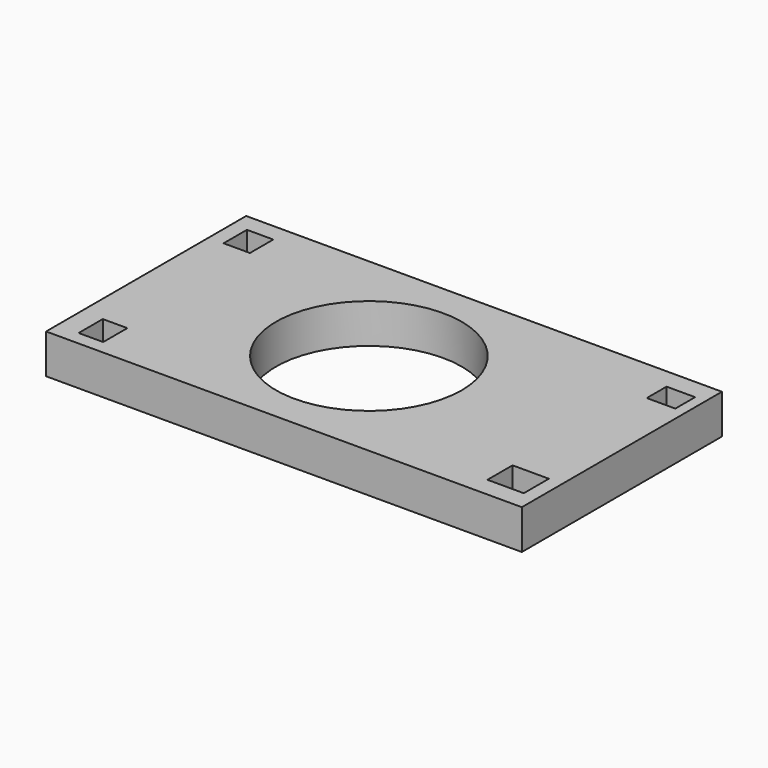
from build123d import *

# Parameters (mm, degrees)
F0_W      = 306.200504303
F0_H      = 160.9693467617
F1_DEPTH  = 25.4
F2_W      = 16.9635862112
F2_H      = 18.7774226069
F2_W_2    = 18.3757990599
F2_H_2    = 15.9212723374
F2_W_3    = 15.8156380057
F2_H_3    = 19.4401964545
F3_DEPTH  = 25.4
F4_W      = 23.3820155263
F4_H      = 20.1737955213
F5_DEPTH  = 25.4
F10_W     = 156.8522006273
F10_H     = 128.1716823578
F10_W_2   = 155.7295322418
F10_H_2   = 9.3674659729
F11_DEPTH = 25.4
F12_R     = 59.7527814568
F13_DEPTH = 25.4


# Not quite as in the source:
# - a feature of the source that left no trace in its solid (it failed there, or was rolled back) is left out


with BuildPart() as f1:
    # F0 (on Top) → F1 (new body)
    with BuildSketch(Plane.XY):
        Rectangle(F0_W, F0_H)
    extrude(amount=F1_DEPTH)

    # F2 (on face) → F3 (cut)
    with BuildSketch(Plane.XY.offset(25.4)):
        with Locations((-134.9064931273, 59.5765523612)):
            Rectangle(F2_W, F2_H)
        with Locations((137.0917782187, 59.4723559916)):
            Rectangle(F2_W_2, F2_H_2)
        with Locations((-131.3789226115, -61.8558935821)):
            Rectangle(F2_W_3, F2_H_3)
    extrude(amount=-F3_DEPTH, mode=Mode.SUBTRACT)

    # F4 (on face) → F5 (cut)
    with BuildSketch(Plane.XY.offset(25.4)):
        with Locations((132.6544694602, -57.8851737082)):
            Rectangle(F4_W, F4_H)
    extrude(amount=-F5_DEPTH, mode=Mode.SUBTRACT)

    # F10 (on Right) → F11 (cut)
    with BuildSketch(Plane.YZ):
        with Locations((274.1180285811, -160.389393568)):
            Rectangle(F10_W, F10_H)
        with Locations((-275.496006012, 285.2313816547)):
            Rectangle(F10_W_2, F10_H_2)
    extrude(amount=-F11_DEPTH, mode=Mode.SUBTRACT)

    # F12 (on face) → F13 (cut)
    with BuildSketch(Plane.XY.offset(25.4)):
        with Locations((-9.737694636, 0)):
            Circle(F12_R)
    extrude(amount=-F13_DEPTH, mode=Mode.SUBTRACT)


solid = f1.part
